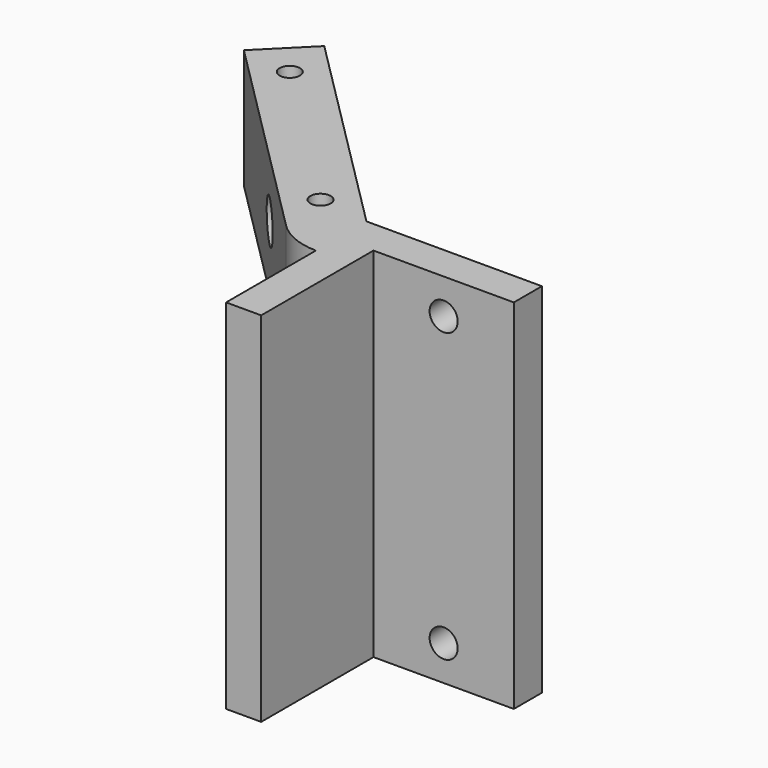
from build123d import *

# Parameters (mm, degrees)
F0_R     = 1.45
F1_DEPTH = 17
F2_DEPTH = 51
F3_R     = 1
F4_DEPTH = 43.4286695297
F3_R_2   = 2.4
F5_DEPTH = 4
F6_SIZE  = 2
F7_R     = 2
F8_DEPTH = 25.001


# Not quite as in the source:
# - a feature names something its author has since deleted; it is built from what else it names


with BuildPart() as f1:
    # F0 (on Top) → F1 (new body)
    with BuildSketch(Plane.XY):
        with BuildLine():
            ThreePointArc((-6.2514946472, 3.0411327703), (-8.8875336165, 9.4050938009), (-6.2514946472, 15.7690548316))
            Line((-6.2514946472, 15.7690548316), (-29.9395718169, 39.4571320014))
            Line((-29.9395718169, 39.4571320014), (-36.3035328476, 33.0931709707))
            Line((-36.3035328476, 33.0931709707), (-6.2514946472, 3.0411327703))
        make_face()
        with Locations((-29.0556883405, 32.2092874942)):
            Circle(F0_R, mode=Mode.SUBTRACT)
        with BuildLine():
            Line((-6.2514946472, 3.0411327703), (0.1124663835, 9.4050938009))
            Line((0.1124663835, 9.4050938009), (-6.2514946472, 15.7690548316))
            ThreePointArc((-6.2514946472, 15.7690548316), (-8.8875336165, 9.4050938009), (-6.2514946472, 3.0411327703))
        make_face()
        with Locations((-7.1353781237, 10.2889772774)):
            Circle(F0_R, mode=Mode.SUBTRACT)
        with BuildLine():
            Line((0.1124663835, 0.4050938009), (0.1124663835, 9.4050938009))
            Line((0.1124663835, 9.4050938009), (-6.2514946472, 3.0411327703))
            ThreePointArc((-6.2514946472, 3.0411327703), (-3.3316845078, 1.0901780083), (0.1124663835, 0.4050938009))
        make_face()
    extrude(amount=-F1_DEPTH)

    # F0 (on Top) → F2 (join)
    with BuildSketch(Plane.XY):
        with BuildLine():
            ThreePointArc((5.1124663835, 1.9217790274), (2.7249524636, 0.7926077208), (0.1124663835, 0.4050938009))
            Line((0.1124663835, 0.4050938009), (0.1124663835, -15.5949061991))
            Line((0.1124663835, -15.5949061991), (5.1124663835, -15.5949061991))
            Line((5.1124663835, -15.5949061991), (5.1124663835, 1.9217790274))
        make_face()
        with BuildLine():
            Line((9.1124663835, 9.4050938009), (0.1124663835, 9.4050938009))
            Line((0.1124663835, 9.4050938009), (0.1124663835, 0.4050938009))
            ThreePointArc((0.1124663835, 0.4050938009), (2.7249524636, 0.7926077208), (5.1124663835, 1.9217790274))
            Line((5.1124663835, 1.9217790274), (5.1124663835, 4.4050938009))
            Line((5.1124663835, 4.4050938009), (7.595781157, 4.4050938009))
            ThreePointArc((7.595781157, 4.4050938009), (8.7249524636, 6.7926077208), (9.1124663835, 9.4050938009))
        make_face()
        with BuildLine():
            Line((25.1124663835, 9.4050938009), (9.1124663835, 9.4050938009))
            ThreePointArc((9.1124663835, 9.4050938009), (8.7249524636, 6.7926077208), (7.595781157, 4.4050938009))
            Line((7.595781157, 4.4050938009), (25.1124663835, 4.4050938009))
            Line((25.1124663835, 4.4050938009), (25.1124663835, 9.4050938009))
        make_face()
    extrude(amount=-F2_DEPTH)

    # F3 (on face) → F4 (cut, through all)
    with BuildSketch(Plane(origin=(4.7587800922, 4.7587800922, 0), x_dir=(-0.7071067812, 0.7071067812, 0), z_dir=(0.7071067812, 0.7071067812, 0))):
        with Locations((23.0708798619, -8)):
            Circle(F3_R)
    extrude(amount=-F4_DEPTH, mode=Mode.SUBTRACT)

    # F3 (on face) → F5 (cut)
    with BuildSketch(Plane(origin=(4.7587800922, 4.7587800922, 0), x_dir=(-0.7071067812, 0.7071067812, 0), z_dir=(0.7071067812, 0.7071067812, 0))):
        with Locations((23.0708798619, -8)):
            Circle(F3_R_2)
        with Locations((23.0708798619, -8)):
            Circle(F3_R, mode=Mode.SUBTRACT)
    extrude(amount=-F5_DEPTH, mode=Mode.SUBTRACT)

    # F6
    f6_edges = [f1.edges().sort_by_distance(p)[0] for p in [
        (-17.21165, 14.001288, -8),
    ]]
    chamfer(f6_edges, length=F6_SIZE)

    # F7 (on face) → F8 (cut, through all)
    with BuildSketch(Plane(origin=(0, 9.4050938009, 0), x_dir=(-1, 0, 0), z_dir=(0, 1, 0))):
        with Locations((-15.1124663835, -5)):
            Circle(F7_R)
        with Locations((-15.1124663835, -46)):
            Circle(F7_R)
    extrude(amount=-F8_DEPTH, mode=Mode.SUBTRACT)


solid = f1.part
